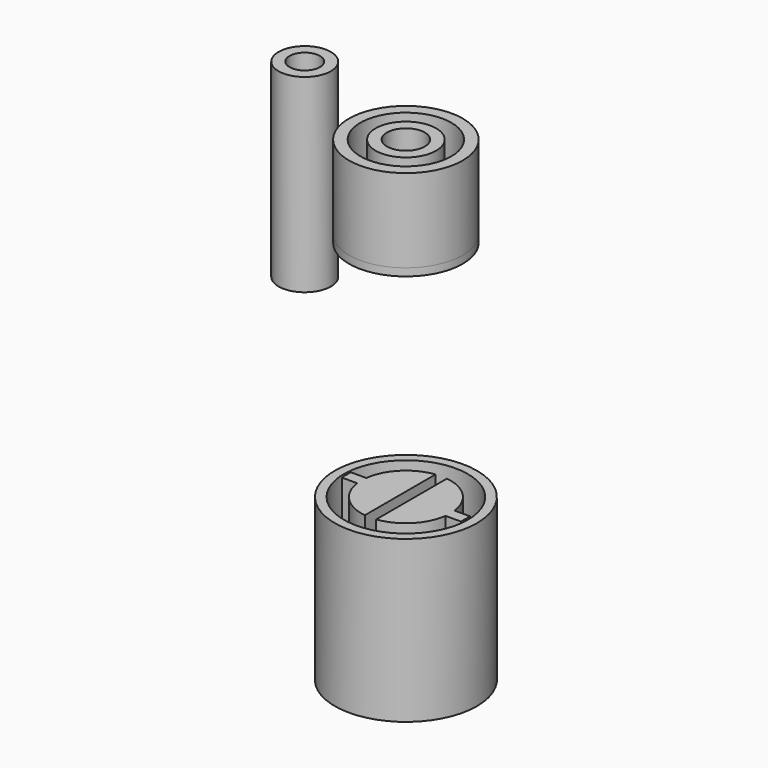
from build123d import *

# Parameters (mm, degrees)
F2_DEPTH  = 19.5
F3_DEPTH  = 1
F4_R      = 9.375
F4_R_2    = 8.175
F4_R_3    = 7.875
F4_R_4    = 4
F5_DEPTH  = 0.75
F6_DEPTH  = 20.5
F8_R      = 7.5
F8_R_2    = 6
F8_R_3    = 4
F9_DEPTH  = 1
F10_DEPTH = 11
F12_DEPTH = 1
F11_R     = 4
F11_R_2   = 2.5
F13_DEPTH = 11
F14_R     = 3.45
F14_R_2   = 2
F15_DEPTH = 25


with BuildPart() as f2:
    # F1 (on Top) → F2 (new body)
    with BuildSketch(Plane.XY):
        with BuildLine():
            Line((-5.8269310104, 0.75), (-7.8392043601, 0.75))
            ThreePointArc((-7.8392043601, 0.75), (-7.875, 0), (-7.8392043601, -0.75))
            Line((-7.8392043601, -0.75), (-5.8269310104, -0.75))
            ThreePointArc((-5.8269310104, -0.75), (-4.1542523395, -4.1542523395), (-0.75, -5.8269310104))
            Line((-0.75, -5.8269310104), (-0.75, 5.8269310104))
            ThreePointArc((-0.75, 5.8269310104), (-4.1542523395, 4.1542523395), (-5.8269310104, 0.75))
        make_face()
    extrude(amount=F2_DEPTH)



with BuildPart() as f2b:
    # F1 (on Top) → F2, piece 2 (new body)
    with BuildSketch(Plane.XY):
        with BuildLine():
            ThreePointArc((7.8392043601, -0.75), (7.8660459996, -0.3754268663), (7.875, 0))
            ThreePointArc((7.875, 0), (7.8660459996, 0.3754268663), (7.8392043601, 0.75))
            Line((7.8392043601, 0.75), (5.8269310104, 0.75))
            ThreePointArc((5.8269310104, 0.75), (4.1542523395, 4.1542523395), (0.75, 5.8269310104))
            Line((0.75, 5.8269310104), (0.75, -5.8269310104))
            ThreePointArc((0.75, -5.8269310104), (4.1542523395, -4.1542523395), (5.8269310104, -0.75))
            Line((5.8269310104, -0.75), (7.8392043601, -0.75))
        make_face()
    extrude(amount=F2_DEPTH)


with BuildPart() as f2_1:
    add(f2.part)

    add(f2b.part)  # F3 merges F2b
    # F1 (on Top) → F3 (join)
    with BuildSketch(Plane.XY):
        with BuildLine():
            Line((5.8269310104, 0.75), (7.8392043601, 0.75))
            ThreePointArc((7.8392043601, 0.75), (0, 7.875), (-7.8392043601, 0.75))
            Line((-7.8392043601, 0.75), (-5.8269310104, 0.75))
            ThreePointArc((-5.8269310104, 0.75), (-4.1542523395, 4.1542523395), (-0.75, 5.8269310104))
            Line((-0.75, 5.8269310104), (-0.75, -5.8269310104))
            ThreePointArc((-0.75, -5.8269310104), (-4.1542523395, -4.1542523395), (-5.8269310104, -0.75))
            Line((-5.8269310104, -0.75), (-7.8392043601, -0.75))
            ThreePointArc((-7.8392043601, -0.75), (0, -7.875), (7.8392043601, -0.75))
            Line((7.8392043601, -0.75), (5.8269310104, -0.75))
            ThreePointArc((5.8269310104, -0.75), (4.1542523395, -4.1542523395), (0.75, -5.8269310104))
            Line((0.75, -5.8269310104), (0.75, 5.8269310104))
            ThreePointArc((0.75, 5.8269310104), (4.1542523395, 4.1542523395), (5.8269310104, 0.75))
        make_face()
        with BuildLine():
            Line((-5.8269310104, 0.75), (-7.8392043601, 0.75))
            ThreePointArc((-7.8392043601, 0.75), (-7.875, 0), (-7.8392043601, -0.75))
            Line((-7.8392043601, -0.75), (-5.8269310104, -0.75))
            ThreePointArc((-5.8269310104, -0.75), (-4.1542523395, -4.1542523395), (-0.75, -5.8269310104))
            Line((-0.75, -5.8269310104), (-0.75, 5.8269310104))
            ThreePointArc((-0.75, 5.8269310104), (-4.1542523395, 4.1542523395), (-5.8269310104, 0.75))
        make_face()
        with BuildLine():
            ThreePointArc((7.8392043601, -0.75), (7.8660459996, -0.3754268663), (7.875, 0))
            ThreePointArc((7.875, 0), (7.8660459996, 0.3754268663), (7.8392043601, 0.75))
            Line((7.8392043601, 0.75), (5.8269310104, 0.75))
            ThreePointArc((5.8269310104, 0.75), (4.1542523395, 4.1542523395), (0.75, 5.8269310104))
            Line((0.75, 5.8269310104), (0.75, -5.8269310104))
            ThreePointArc((0.75, -5.8269310104), (4.1542523395, -4.1542523395), (5.8269310104, -0.75))
            Line((5.8269310104, -0.75), (7.8392043601, -0.75))
        make_face()
    extrude(amount=-F3_DEPTH)


with BuildPart() as f5:
    # F4 (on face) → F5 (new body)
    with BuildSketch(Plane(origin=(0, 0, -1), x_dir=(1, 0, 0), z_dir=(0, 0, -1))):
        Circle(F4_R)
        Circle(F4_R_2, mode=Mode.SUBTRACT)
        Circle(F4_R_2)
        Circle(F4_R_3, mode=Mode.SUBTRACT)
        Circle(F4_R_3)
        Circle(F4_R_4, mode=Mode.SUBTRACT)
    extrude(amount=F5_DEPTH)

    # F4 (on face) → F6 (join)
    with BuildSketch(Plane(origin=(0, 0, -1), x_dir=(1, 0, 0), z_dir=(0, 0, -1))):
        Circle(F4_R)
        Circle(F4_R_2, mode=Mode.SUBTRACT)
    extrude(amount=-F6_DEPTH)


with BuildPart() as f9:
    # F8 (on offset) → F9 (new body)
    with BuildSketch(Plane.XY.offset(50)):
        Circle(F8_R)
        Circle(F8_R_2, mode=Mode.SUBTRACT)
        Circle(F8_R_2)
        Circle(F8_R_3, mode=Mode.SUBTRACT)
    extrude(amount=-F9_DEPTH)

    # F8 (on offset) → F10 (join)
    with BuildSketch(Plane.XY.offset(50)):
        Circle(F8_R)
        Circle(F8_R_2, mode=Mode.SUBTRACT)
    extrude(amount=F10_DEPTH)


with BuildPart() as f12:
    # F8 (on offset) → F12 (new body)
    with BuildSketch(Plane.XY.offset(50)):
        Circle(F8_R_2)
        Circle(F8_R_3, mode=Mode.SUBTRACT)
        Circle(F8_R_3)
    extrude(amount=F12_DEPTH)

    # F11 (on offset) → F13 (join)
    with BuildSketch(Plane.XY.offset(50)):
        Circle(F11_R)
        Circle(F11_R_2, mode=Mode.SUBTRACT)
    extrude(amount=F13_DEPTH)


with BuildPart() as f15:
    # F14 (on Top) → F15 (new body)
    with BuildSketch(Plane.XY):
        with Locations((-62.1994845569, 61.0717199743)):
            Circle(F14_R)
        with Locations((-62.1994845569, 61.0717199743)):
            Circle(F14_R_2, mode=Mode.SUBTRACT)
    extrude(amount=F15_DEPTH)


solid = Compound([f2_1.part, f5.part, f9.part, f12.part, f15.part])
